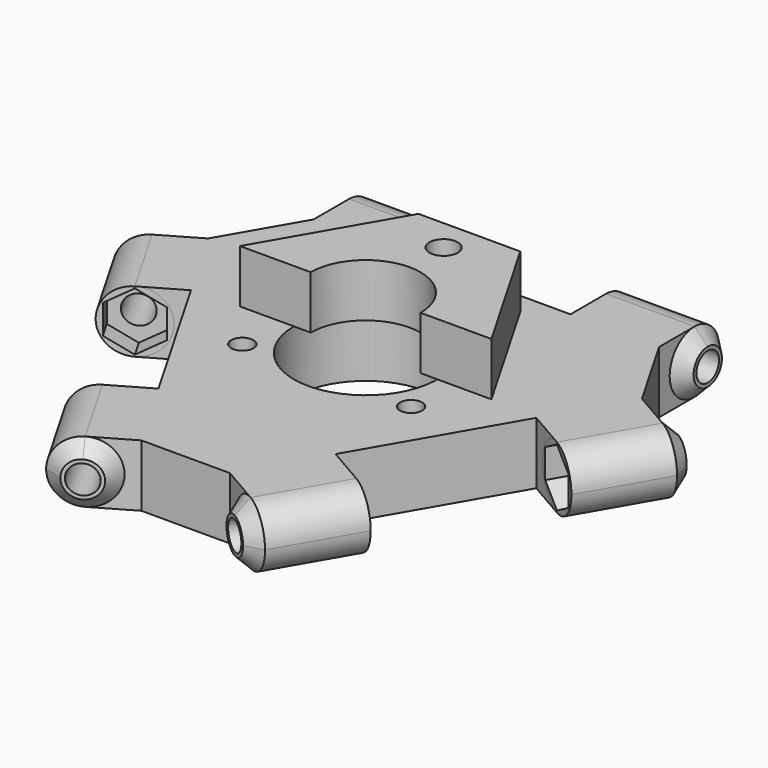
from build123d import *

# Parameters (mm, degrees)
F5_R           = 1.25
F5_R_2         = 1.6
F6_DEPTH       = 7
F7_DEPTH       = 6
F8_R           = 3.49999
F9_R           = 1.6
F10_DEPTH      = 11.5
F10_DEPTH_BACK = 30.5
F11_DEPTH      = 19
F12_DEPTH      = 2.3
F12_DEPTH_BACK = 21.3
F13_DEPTH      = 10
F13_DEPTH_BACK = 29
F14_R          = 1.6
F15_DEPTH      = 11.5
F15_DEPTH_BACK = 30.5
F16_DEPTH      = 19
F17_DEPTH      = 2.3
F17_DEPTH_BACK = 21.3
F18_DEPTH      = 10
F18_DEPTH_BACK = 29
F19_R          = 1.6
F20_DEPTH      = 11.5
F20_DEPTH_BACK = 30.5
F21_DEPTH      = 19
F22_DEPTH      = 2.3
F22_DEPTH_BACK = 21.3
F23_DEPTH      = 10
F23_DEPTH_BACK = 29
F24_C1_SIZE    = 1.4999
F24_C2_SIZE    = 1.4999
F24_C3_SIZE    = 1.4999
F24_C4_SIZE    = 1.4996
F24_C5_SIZE    = 1.4999
F24_C6_SIZE    = 1.4999


# Not quite as in the source:
# - a fillet or chamfer is up to 0.001 mm smaller than in the source, because OpenCascade refuses the exact size
# - a feature names something its author has since deleted; it is built from what else it names


with BuildPart() as f6:
    # F5 (on Top) → F6 (new body)
    with BuildSketch(Plane.XY):
        Polygon((9.5, 17.0318329411), (-9.5, 17.0318329411), (-9.5, 25.5318329411), (-19.5, 25.5318329411), (-19.5, 17.0318329411), (-24.5, 8.3715789032), (-31.8612159322, 4.1215789032), (-26.8612159322, -4.5386751346), (-19.5, -0.2886751346), (-10, -16.7431578065), (-17.3612159322, -20.9931578065), (-12.3612159322, -29.6534118443), (-5, -25.4034118443), (5, -25.4034118443), (12.3612159322, -29.6534118443), (17.3612159322, -20.9931578065), (10, -16.7431578065), (19.5, -0.2886751346), (26.8612159322, -4.5386751346), (31.8612159322, 4.1215789032), (24.5, 8.3715789032), (19.5, 17.0318329411), (19.5, 25.5318329411), (9.5, 25.5318329411), align=None)
        with Locations((-9.5262794416, -5.5)):
            Circle(F5_R, mode=Mode.SUBTRACT)
        with Locations((9.5262794416, -5.5)):
            Circle(F5_R, mode=Mode.SUBTRACT)
        with BuildLine():
            Line((14.2, 0), (8.1, 0))
            ThreePointArc((8.1, 0), (0, -8.1), (-8.1, 0))
            Line((-8.1, 0), (-14.2, 0))
            Line((-14.2, 0), (-5.75, 14.635829324))
            Line((-5.75, 14.635829324), (5.75, 14.635829324))
            Line((5.75, 14.635829324), (14.2, 0))
        make_face(mode=Mode.SUBTRACT)
        with BuildLine():
            ThreePointArc((-8.1, 0), (0, 8.1), (8.1, 0))
            Line((8.1, 0), (14.2, 0))
            Line((14.2, 0), (5.75, 14.635829324))
            Line((5.75, 14.635829324), (-5.75, 14.635829324))
            Line((-5.75, 14.635829324), (-14.2, 0))
            Line((-14.2, 0), (-8.1, 0))
        make_face()
        with Locations((0, 11)):
            Circle(F5_R_2, mode=Mode.SUBTRACT)
        with Locations((0, 11)):
            Circle(F5_R_2)
        with Locations((0, 11)):
            Circle(F5_R, mode=Mode.SUBTRACT)
    extrude(amount=-F6_DEPTH)

    # F8 (radius 3.5 in the source; OpenCascade refuses exactly that, so slightly less here)
    f8_edges = [f6.edges().sort_by_distance(p)[0] for p in [
        (14.861216, -25.323285, -7),
        (29.361216, -0.208548, -7),
        (14.861216, -25.323285, 0),
        (29.361216, -0.208548, 0),
        (-14.861216, -25.323285, -7),
        (-14.861216, -25.323285, 0),
        (-29.361216, -0.208548, 0),
        (-29.361216, -0.208548, -7),
        (14.5, 25.531833, -7),
        (-14.5, 25.531833, -7),
        (14.5, 25.531833, 0),
        (-14.5, 25.531833, 0),
    ]]
    fillet(f8_edges, radius=F8_R)

    # F9 (on face) → F10 (join, two sides)
    with BuildSketch(Plane(origin=(4.75, 8.227241336, 0), x_dir=(0.8660254038, -0.5, 0), z_dir=(-0.5, -0.8660254038, 0))) as f10_sk:
        with BuildLine():
            ThreePointArc((22.0318429411, -7), (24.5067102108, -5.9748701986), (25.5318329411, -3.5))
            ThreePointArc((25.5318329411, -3.5), (24.5067102108, -1.0251298014), (22.0318429411, 0))
            ThreePointArc((22.0318429411, 0), (18.5318329411, -3.5), (22.0318429411, -7))
        make_face()
        Polygon((19.1818329411, -1.8545517328), (22.0318329411, -0.2091034656), (24.8818329411, -1.8545517328), (24.8818329411, -5.1454482672), (22.0318329411, -6.7908965344), (19.1818329411, -5.1454482672), align=None, mode=Mode.SUBTRACT)
        Polygon((24.8818329411, -1.8545517328), (22.0318329411, -0.2091034656), (19.1818329411, -1.8545517328), (19.1818329411, -5.1454482672), (22.0318329411, -6.7908965344), (24.8818329411, -5.1454482672), align=None)
        with Locations((22.0318329411, -3.5)):
            Circle(F9_R, mode=Mode.SUBTRACT)
    extrude(amount=-F10_DEPTH)
    extrude(f10_sk.sketch, amount=F10_DEPTH_BACK)

    # F9 (on face) → F11 (cut)
    with BuildSketch(Plane(origin=(4.75, 8.227241336, 0), x_dir=(0.8660254038, -0.5, 0), z_dir=(-0.5, -0.8660254038, 0))):
        with BuildLine():
            ThreePointArc((22.0318429411, -7), (24.5067102108, -5.9748701986), (25.5318329411, -3.5))
            ThreePointArc((25.5318329411, -3.5), (24.5067102108, -1.0251298014), (22.0318429411, 0))
            ThreePointArc((22.0318429411, 0), (18.5318329411, -3.5), (22.0318429411, -7))
        make_face()
        Polygon((19.1818329411, -1.8545517328), (22.0318329411, -0.2091034656), (24.8818329411, -1.8545517328), (24.8818329411, -5.1454482672), (22.0318329411, -6.7908965344), (19.1818329411, -5.1454482672), align=None, mode=Mode.SUBTRACT)
        Polygon((24.8818329411, -1.8545517328), (22.0318329411, -0.2091034656), (19.1818329411, -1.8545517328), (19.1818329411, -5.1454482672), (22.0318329411, -6.7908965344), (24.8818329411, -5.1454482672), align=None)
        with Locations((22.0318329411, -3.5)):
            Circle(F9_R, mode=Mode.SUBTRACT)
    extrude(amount=F11_DEPTH, mode=Mode.SUBTRACT)

    # F9 (on face) → F12 (cut, two sides)
    with BuildSketch(Plane(origin=(4.75, 8.227241336, 0), x_dir=(0.8660254038, -0.5, 0), z_dir=(-0.5, -0.8660254038, 0))) as f12_sk:
        Polygon((24.8818329411, -1.8545517328), (22.0318329411, -0.2091034656), (19.1818329411, -1.8545517328), (19.1818329411, -5.1454482672), (22.0318329411, -6.7908965344), (24.8818329411, -5.1454482672), align=None)
        with Locations((22.0318329411, -3.5)):
            Circle(F9_R, mode=Mode.SUBTRACT)
    extrude(amount=-F12_DEPTH, mode=Mode.SUBTRACT)
    extrude(f12_sk.sketch, amount=F12_DEPTH_BACK, mode=Mode.SUBTRACT)

    # F9 (on face) → F13 (cut, two sides)
    with BuildSketch(Plane(origin=(4.75, 8.227241336, 0), x_dir=(0.8660254038, -0.5, 0), z_dir=(-0.5, -0.8660254038, 0))) as f13_sk:
        with Locations((22.0318329411, -3.5)):
            Circle(F9_R)
    extrude(amount=-F13_DEPTH, mode=Mode.SUBTRACT)
    extrude(f13_sk.sketch, amount=F13_DEPTH_BACK, mode=Mode.SUBTRACT)

    # F14 (on face) → F15 (join, two sides)
    with BuildSketch(Plane(origin=(4.75, -8.227241336, 0), x_dir=(-0.8660254038, -0.5, 0), z_dir=(-0.5, 0.8660254038, 0))) as f15_sk:
        with BuildLine():
            ThreePointArc((22.0318429411, -7), (24.5067102108, -5.9748701986), (25.5318329411, -3.5))
            ThreePointArc((25.5318329411, -3.5), (24.5067102108, -1.0251298014), (22.0318429411, 0))
            ThreePointArc((22.0318429411, 0), (18.5318329411, -3.5), (22.0318429411, -7))
        make_face()
        Polygon((19.1818329411, -1.8545517328), (22.0318329411, -0.2091034656), (24.8818329411, -1.8545517328), (24.8818329411, -5.1454482672), (22.0318329411, -6.7908965344), (19.1818329411, -5.1454482672), align=None, mode=Mode.SUBTRACT)
        Polygon((24.8818329411, -1.8545517328), (22.0318329411, -0.2091034656), (19.1818329411, -1.8545517328), (19.1818329411, -5.1454482672), (22.0318329411, -6.7908965344), (24.8818329411, -5.1454482672), align=None)
        with Locations((22.0318329411, -3.5)):
            Circle(F14_R, mode=Mode.SUBTRACT)
    extrude(amount=-F15_DEPTH)
    extrude(f15_sk.sketch, amount=F15_DEPTH_BACK)

    # F14 (on face) → F16 (cut)
    with BuildSketch(Plane(origin=(4.75, -8.227241336, 0), x_dir=(-0.8660254038, -0.5, 0), z_dir=(-0.5, 0.8660254038, 0))):
        with BuildLine():
            ThreePointArc((22.0318429411, -7), (24.5067102108, -5.9748701986), (25.5318329411, -3.5))
            ThreePointArc((25.5318329411, -3.5), (24.5067102108, -1.0251298014), (22.0318429411, 0))
            ThreePointArc((22.0318429411, 0), (18.5318329411, -3.5), (22.0318429411, -7))
        make_face()
        Polygon((19.1818329411, -1.8545517328), (22.0318329411, -0.2091034656), (24.8818329411, -1.8545517328), (24.8818329411, -5.1454482672), (22.0318329411, -6.7908965344), (19.1818329411, -5.1454482672), align=None, mode=Mode.SUBTRACT)
        Polygon((24.8818329411, -1.8545517328), (22.0318329411, -0.2091034656), (19.1818329411, -1.8545517328), (19.1818329411, -5.1454482672), (22.0318329411, -6.7908965344), (24.8818329411, -5.1454482672), align=None)
        with Locations((22.0318329411, -3.5)):
            Circle(F14_R, mode=Mode.SUBTRACT)
    extrude(amount=F16_DEPTH, mode=Mode.SUBTRACT)

    # F14 (on face) → F17 (cut, two sides)
    with BuildSketch(Plane(origin=(4.75, -8.227241336, 0), x_dir=(-0.8660254038, -0.5, 0), z_dir=(-0.5, 0.8660254038, 0))) as f17_sk:
        Polygon((24.8818329411, -1.8545517328), (22.0318329411, -0.2091034656), (19.1818329411, -1.8545517328), (19.1818329411, -5.1454482672), (22.0318329411, -6.7908965344), (24.8818329411, -5.1454482672), align=None)
        with Locations((22.0318329411, -3.5)):
            Circle(F14_R, mode=Mode.SUBTRACT)
    extrude(amount=-F17_DEPTH, mode=Mode.SUBTRACT)
    extrude(f17_sk.sketch, amount=F17_DEPTH_BACK, mode=Mode.SUBTRACT)

    # F14 (on face) → F18 (cut, two sides)
    with BuildSketch(Plane(origin=(4.75, -8.227241336, 0), x_dir=(-0.8660254038, -0.5, 0), z_dir=(-0.5, 0.8660254038, 0))) as f18_sk:
        with Locations((22.0318329411, -3.5)):
            Circle(F14_R)
    extrude(amount=-F18_DEPTH, mode=Mode.SUBTRACT)
    extrude(f18_sk.sketch, amount=F18_DEPTH_BACK, mode=Mode.SUBTRACT)

    # F19 (on face) → F20 (join, two sides)
    with BuildSketch(Plane.YZ.offset(-9.5)) as f20_sk:
        with BuildLine():
            ThreePointArc((22.0318429411, -7), (24.5067102108, -5.9748701986), (25.5318329411, -3.5))
            ThreePointArc((25.5318329411, -3.5), (24.5067102108, -1.0251298014), (22.0318429411, 0))
            ThreePointArc((22.0318429411, 0), (18.5318329411, -3.5), (22.0318429411, -7))
        make_face()
        Polygon((19.1818329411, -1.8545517328), (22.0318329411, -0.2091034656), (24.8818329411, -1.8545517328), (24.8818329411, -5.1454482672), (22.0318329411, -6.7908965344), (19.1818329411, -5.1454482672), align=None, mode=Mode.SUBTRACT)
        Polygon((24.8818329411, -1.8545517328), (22.0318329411, -0.2091034656), (19.1818329411, -1.8545517328), (19.1818329411, -5.1454482672), (22.0318329411, -6.7908965344), (24.8818329411, -5.1454482672), align=None)
        with Locations((22.0318329411, -3.5)):
            Circle(F19_R, mode=Mode.SUBTRACT)
    extrude(amount=-F20_DEPTH)
    extrude(f20_sk.sketch, amount=F20_DEPTH_BACK)

    # F19 (on face) → F21 (cut)
    with BuildSketch(Plane.YZ.offset(-9.5)):
        with BuildLine():
            ThreePointArc((22.0318429411, -7), (24.5067102108, -5.9748701986), (25.5318329411, -3.5))
            ThreePointArc((25.5318329411, -3.5), (24.5067102108, -1.0251298014), (22.0318429411, 0))
            ThreePointArc((22.0318429411, 0), (18.5318329411, -3.5), (22.0318429411, -7))
        make_face()
        Polygon((19.1818329411, -1.8545517328), (22.0318329411, -0.2091034656), (24.8818329411, -1.8545517328), (24.8818329411, -5.1454482672), (22.0318329411, -6.7908965344), (19.1818329411, -5.1454482672), align=None, mode=Mode.SUBTRACT)
        Polygon((24.8818329411, -1.8545517328), (22.0318329411, -0.2091034656), (19.1818329411, -1.8545517328), (19.1818329411, -5.1454482672), (22.0318329411, -6.7908965344), (24.8818329411, -5.1454482672), align=None)
        with Locations((22.0318329411, -3.5)):
            Circle(F19_R, mode=Mode.SUBTRACT)
    extrude(amount=F21_DEPTH, mode=Mode.SUBTRACT)

    # F19 (on face) → F22 (cut, two sides)
    with BuildSketch(Plane.YZ.offset(-9.5)) as f22_sk:
        Polygon((24.8818329411, -1.8545517328), (22.0318329411, -0.2091034656), (19.1818329411, -1.8545517328), (19.1818329411, -5.1454482672), (22.0318329411, -6.7908965344), (24.8818329411, -5.1454482672), align=None)
        with Locations((22.0318329411, -3.5)):
            Circle(F19_R, mode=Mode.SUBTRACT)
    extrude(amount=-F22_DEPTH, mode=Mode.SUBTRACT)
    extrude(f22_sk.sketch, amount=F22_DEPTH_BACK, mode=Mode.SUBTRACT)

    # F19 (on face) → F23 (cut, two sides)
    with BuildSketch(Plane.YZ.offset(-9.5)) as f23_sk:
        with Locations((22.0318329411, -3.5)):
            Circle(F19_R)
    extrude(amount=-F23_DEPTH, mode=Mode.SUBTRACT)
    extrude(f23_sk.sketch, amount=F23_DEPTH_BACK, mode=Mode.SUBTRACT)

    # F24: chamfer of 1.5 on 6 edges, made by hand

    # F24_c1 (size 1.5 in the source; OpenCascade refuses exactly that, so slightly less here)
    f24_c1_edges = [f6.edges().sort_by_distance(p)[0] for p in [
        (-21, 22.0318229411, 0),
    ]]
    chamfer(f24_c1_edges, length=F24_C1_SIZE)

    # F24_c2 (size 1.5 in the source; OpenCascade refuses exactly that, so slightly less here)
    f24_c2_edges = [f6.edges().sort_by_distance(p)[0] for p in [
        (21, 22.0318229411, 0),
    ]]
    chamfer(f24_c2_edges, length=F24_C2_SIZE)

    # F24_c3 (size 1.5 in the source; OpenCascade refuses exactly that, so slightly less here)
    f24_c3_edges = [f6.edges().sort_by_distance(p)[0] for p in [
        (29.5801183587, 7.1706220089, 0),
    ]]
    chamfer(f24_c3_edges, length=F24_C3_SIZE)

    # F24_c4 (size 1.5 in the source; OpenCascade refuses exactly that, so slightly less here)
    f24_c4_edges = [f6.edges().sort_by_distance(p)[0] for p in [
        (8.5801183587, -29.20244495, 0),
    ]]
    chamfer(f24_c4_edges, length=F24_C4_SIZE)

    # F24_c5 (size 1.5 in the source; OpenCascade refuses exactly that, so slightly less here)
    f24_c5_edges = [f6.edges().sort_by_distance(p)[0] for p in [
        (-8.5801183587, -29.20244495, 0),
    ]]
    chamfer(f24_c5_edges, length=F24_C5_SIZE)

    # F24_c6 (size 1.5 in the source; OpenCascade refuses exactly that, so slightly less here)
    f24_c6_edges = [f6.edges().sort_by_distance(p)[0] for p in [
        (-29.5801183587, 7.1706220089, 0),
    ]]
    chamfer(f24_c6_edges, length=F24_C6_SIZE)


with BuildPart() as f7:
    # F5 (on Top) → F7 (new body)
    with BuildSketch(Plane.XY):
        with BuildLine():
            ThreePointArc((-8.1, 0), (0, 8.1), (8.1, 0))
            Line((8.1, 0), (14.2, 0))
            Line((14.2, 0), (5.75, 14.635829324))
            Line((5.75, 14.635829324), (-5.75, 14.635829324))
            Line((-5.75, 14.635829324), (-14.2, 0))
            Line((-14.2, 0), (-8.1, 0))
        make_face()
        with Locations((0, 11)):
            Circle(F5_R_2, mode=Mode.SUBTRACT)
        with BuildLine():
            Line((6.2, 0), (8.1, 0))
            ThreePointArc((8.1, 0), (0, 8.1), (-8.1, 0))
            Line((-8.1, 0), (-6.2, 0))
            ThreePointArc((-6.2, 0), (0, 6.2), (6.2, 0))
        make_face()
    extrude(amount=F7_DEPTH)


solid = Compound([f6.part, f7.part])
